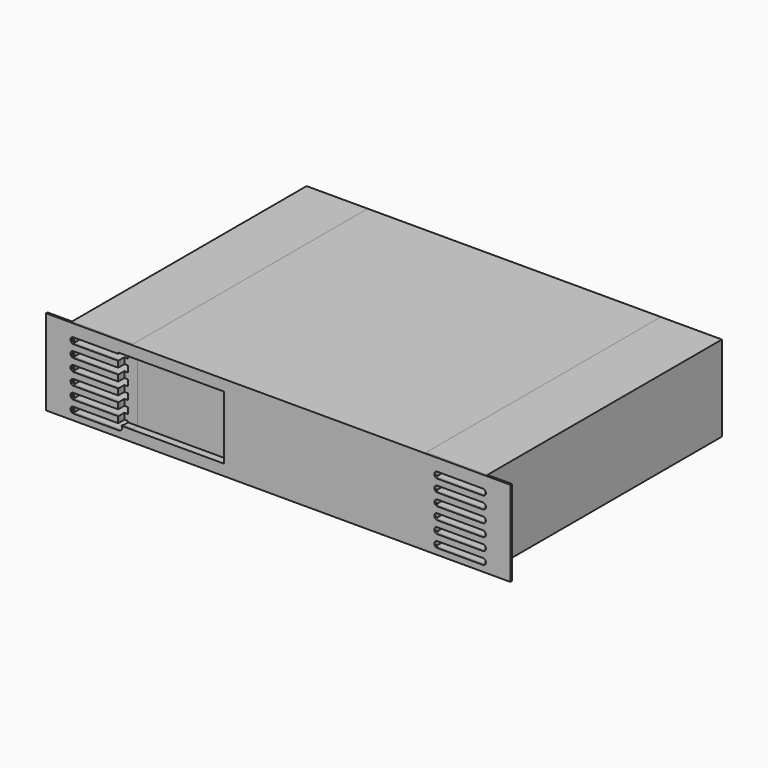
from build123d import *

# Parameters (mm, degrees)
F0_W      = 304.8
F0_H      = 304.8
F1_DEPTH  = 88.9
F2_W      = 88.9
F2_H      = 88.9
F2_W_2    = 304.8
F3_DEPTH  = 2
F5_DEPTH  = 254
F7_DEPTH  = 2.001
F9_DEPTH  = 304.801
F10_DEPTH = 304.8
F11_W     = 110
F11_H     = 66
F12_DEPTH = 8


with BuildPart() as f1:
    # F0 (on Top) → F1 (new body)
    with BuildSketch(Plane.XY):
        Rectangle(F0_W, F0_H)
    extrude(amount=F1_DEPTH)

    # F2 (on face) → F3 (join)
    with BuildSketch(Plane.XZ.offset(152.4)):
        with Locations((-196.85, 44.45)):
            Rectangle(F2_W, F2_H)
        with Locations((0, 44.45)):
            Rectangle(F2_W_2, F2_H)
        with Locations((196.85, 44.45)):
            Rectangle(F2_W, F2_H)
    extrude(amount=F3_DEPTH)

    # F6 (on face) → F7 (cut, through all)
    with BuildSketch(Plane(origin=(0, -152.4, 0), x_dir=(-1, 0, 0), z_dir=(0, 1, 0))):
        with BuildLine():
            Line((-165.575, 76.2), (-212.725, 76.2))
            ThreePointArc((-212.725, 76.2), (-215.9, 73.025), (-212.725, 69.85))
            Line((-212.725, 69.85), (-165.575, 69.85))
            ThreePointArc((-165.575, 69.85), (-162.4, 73.025), (-165.575, 76.2))
        make_face()
        with BuildLine():
            Line((-165.575, 63.5), (-212.725, 63.5))
            ThreePointArc((-212.725, 63.5), (-215.9, 60.325), (-212.725, 57.15))
            Line((-212.725, 57.15), (-165.575, 57.15))
            ThreePointArc((-165.575, 57.15), (-162.4, 60.325), (-165.575, 63.5))
        make_face()
        with BuildLine():
            Line((-165.575, 50.8), (-212.725, 50.8))
            ThreePointArc((-212.725, 50.8), (-215.9, 47.625), (-212.725, 44.45))
            Line((-212.725, 44.45), (-165.575, 44.45))
            ThreePointArc((-165.575, 44.45), (-162.4, 47.625), (-165.575, 50.8))
        make_face()
        with BuildLine():
            Line((-165.575, 38.1), (-212.725, 38.1))
            ThreePointArc((-212.725, 38.1), (-215.9, 34.925), (-212.725, 31.75))
            Line((-212.725, 31.75), (-165.575, 31.75))
            ThreePointArc((-165.575, 31.75), (-162.4, 34.925), (-165.575, 38.1))
        make_face()
        with BuildLine():
            Line((-165.575, 25.4), (-212.725, 25.4))
            ThreePointArc((-212.725, 25.4), (-215.9, 22.225), (-212.725, 19.05))
            Line((-212.725, 19.05), (-165.575, 19.05))
            ThreePointArc((-165.575, 19.05), (-162.4, 22.225), (-165.575, 25.4))
        make_face()
        with BuildLine():
            Line((-165.575, 12.7), (-212.725, 12.7))
            ThreePointArc((-212.725, 12.7), (-215.9, 9.525), (-212.725, 6.35))
            Line((-212.725, 6.35), (-165.575, 6.35))
            ThreePointArc((-165.575, 6.35), (-162.4, 9.525), (-165.575, 12.7))
        make_face()
        with BuildLine():
            ThreePointArc((212.725, 31.75), (215.9, 34.925), (212.725, 38.1))
            Line((212.725, 38.1), (165.575, 38.1))
            ThreePointArc((165.575, 38.1), (162.4, 34.925), (165.575, 31.75))
            Line((165.575, 31.75), (212.725, 31.75))
        make_face()
        with BuildLine():
            Line((165.575, 6.35), (212.725, 6.35))
            ThreePointArc((212.725, 6.35), (215.9, 9.525), (212.725, 12.7))
            Line((212.725, 12.7), (165.575, 12.7))
            ThreePointArc((165.575, 12.7), (162.4, 9.525), (165.575, 6.35))
        make_face()
        with BuildLine():
            ThreePointArc((165.575, 50.8), (162.4, 47.625), (165.575, 44.45))
            Line((165.575, 44.45), (212.725, 44.45))
            ThreePointArc((212.725, 44.45), (215.9, 47.625), (212.725, 50.8))
            Line((212.725, 50.8), (165.575, 50.8))
        make_face()
        with BuildLine():
            ThreePointArc((165.575, 63.5), (162.4, 60.325), (165.575, 57.15))
            Line((165.575, 57.15), (212.725, 57.15))
            ThreePointArc((212.725, 57.15), (215.9, 60.325), (212.725, 63.5))
            Line((212.725, 63.5), (165.575, 63.5))
        make_face()
        with BuildLine():
            ThreePointArc((212.725, 69.85), (215.9, 73.025), (212.725, 76.2))
            Line((212.725, 76.2), (165.575, 76.2))
            ThreePointArc((165.575, 76.2), (162.4, 73.025), (165.575, 69.85))
            Line((165.575, 69.85), (212.725, 69.85))
        make_face()
        with BuildLine():
            Line((165.575, 19.05), (212.725, 19.05))
            ThreePointArc((212.725, 19.05), (215.9, 22.225), (212.725, 25.4))
            Line((212.725, 25.4), (165.575, 25.4))
            ThreePointArc((165.575, 25.4), (162.4, 22.225), (165.575, 19.05))
        make_face()
    extrude(amount=-F7_DEPTH, mode=Mode.SUBTRACT)


with BuildPart() as f5:
    # F4 (on face) → F5 (new body)
    with BuildSketch(Plane(origin=(0, -152.4, 0), x_dir=(-1, 0, 0), z_dir=(0, 1, 0))):
        Polygon((-152.4, 0), (-152.4, 88.9), (-162.4, 88.9), (-162.4, 82.55), (-215.9, 82.55), (-215.9, 76.2), (-162.4, 76.2), (-162.4, 69.85), (-215.9, 69.85), (-215.9, 63.5), (-162.4, 63.5), (-162.4, 57.15), (-215.9, 57.15), (-215.9, 50.8), (-162.4, 50.8), (-162.4, 44.45), (-215.9, 44.45), (-215.9, 38.1), (-162.4, 38.1), (-162.4, 31.75), (-215.9, 31.75), (-215.9, 25.4), (-162.4, 25.4), (-162.4, 19.05), (-215.9, 19.05), (-215.9, 12.7), (-162.4, 12.7), (-162.4, 6.35), (-215.9, 6.35), (-215.9, 0), (-162.4, 0), align=None)
    extrude(amount=F5_DEPTH)


with BuildPart() as f5b:
    # F4 (on face) → F5, piece 2 (new body)
    with BuildSketch(Plane(origin=(0, -152.4, 0), x_dir=(-1, 0, 0), z_dir=(0, 1, 0))):
        Polygon((215.9, 63.5), (215.9, 69.85), (162.4, 69.85), (162.4, 76.2), (215.9, 76.2), (215.9, 82.55), (162.4, 82.55), (162.4, 88.9), (152.4, 88.9), (152.4, 0), (162.4, 0), (215.9, 0), (215.9, 6.35), (162.4, 6.35), (162.4, 12.7), (215.9, 12.7), (215.9, 19.05), (162.4, 19.05), (162.4, 25.4), (215.9, 25.4), (215.9, 31.75), (162.4, 31.75), (162.4, 38.1), (215.9, 38.1), (215.9, 44.45), (162.4, 44.45), (162.4, 50.8), (215.9, 50.8), (215.9, 57.15), (162.4, 57.15), (162.4, 63.5), align=None)
    extrude(amount=F5_DEPTH)


with BuildPart() as f9_tool:
    # F8 (on face) → F9 (new body, through all)
    with BuildSketch(Plane(origin=(0, -152.4, 0), x_dir=(-1, 0, 0), z_dir=(0, 1, 0))):
        Polygon((-152.4, 86.9), (-152.4, 88.9), (-215.9, 88.9), (-215.9, 0), (-152.4, 0), (-152.4, 2), (-213.9, 2), (-213.9, 86.9), align=None)
        Polygon((215.9, 88.9), (152.4, 88.9), (152.4, 86.9), (213.9, 86.9), (213.9, 2), (152.4, 2), (152.4, 0), (215.9, 0), align=None)
    extrude(amount=F9_DEPTH)


with BuildPart() as f5_1:
    add(f5.part)

    # F9: cut by f9_tool
    add(f9_tool.part, mode=Mode.SUBTRACT)


with BuildPart() as f5b_1:
    add(f5b.part)

    # F9: cut by f9_tool
    add(f9_tool.part, mode=Mode.SUBTRACT)


with BuildPart() as f10:
    # F8 (on face) → F10 (new body)
    with BuildSketch(Plane(origin=(0, -152.4, 0), x_dir=(-1, 0, 0), z_dir=(0, 1, 0))):
        Polygon((-152.4, 86.9), (-152.4, 88.9), (-215.9, 88.9), (-215.9, 0), (-152.4, 0), (-152.4, 2), (-213.9, 2), (-213.9, 86.9), align=None)
    extrude(amount=F10_DEPTH)


with BuildPart() as f10b:
    # F8 (on face) → F10, piece 2 (new body)
    with BuildSketch(Plane(origin=(0, -152.4, 0), x_dir=(-1, 0, 0), z_dir=(0, 1, 0))):
        Polygon((215.9, 88.9), (152.4, 88.9), (152.4, 86.9), (213.9, 86.9), (213.9, 2), (152.4, 2), (152.4, 0), (215.9, 0), align=None)
    extrude(amount=F10_DEPTH)


with BuildPart() as f12_tool:
    # F11 (on face) → F12 (new body)
    with BuildSketch(Plane.XZ.offset(154.4)):
        with Locations((-111.3, 44.45)):
            Rectangle(F11_W, F11_H)
    extrude(amount=-F12_DEPTH)


with BuildPart() as f1_1:
    add(f1.part)

    # F12: cut by f12_tool
    add(f12_tool.part, mode=Mode.SUBTRACT)


with BuildPart() as f5b_2:
    add(f5b_1.part)

    # F12: cut by f12_tool
    add(f12_tool.part, mode=Mode.SUBTRACT)


solid = Compound([f5_1.part, f10.part, f10b.part, f1_1.part, f5b_2.part])
